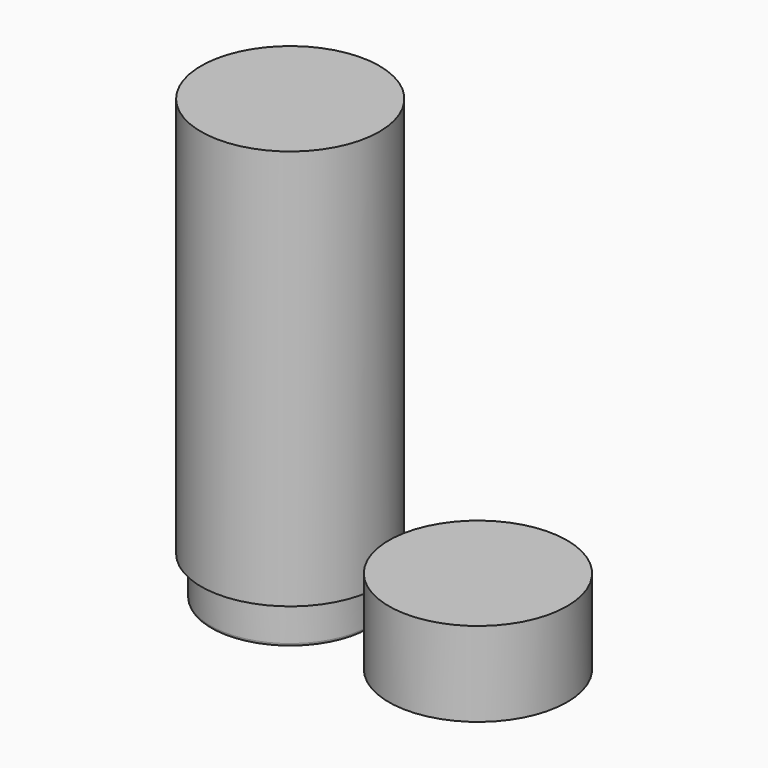
from build123d import *

# Parameters (mm, degrees)
F0_R      = 25.5
F0_R_2    = 22.5
F0_R_3    = 17.5
F1_DEPTH  = 141
F2_DEPTH  = 136
F3_DEPTH  = 66
F5_R      = 1
F6_R      = 1
F7_R      = 1
F8_R      = 28.5
F8_R_2    = 25.5
F8_R_3    = 22.5
F9_DEPTH  = 27
F10_DEPTH = 22
F11_DEPTH = 12
F12_R     = 2
F13_R     = 1
F14_R     = 28.5
F14_R_2   = 25.5
F15_DEPTH = 128


# Not quite as in the source:
# - a fillet or chamfer that OpenCascade refuses, or shapes differently, is made with other operations: its cross-section is extruded or revolved along the edge and cut away or added


with BuildPart() as f1:
    # F0 (on Top) → F1 (new body)
    with BuildSketch(Plane.XY):
        Circle(F0_R)
        Circle(F0_R_2, mode=Mode.SUBTRACT)
        Circle(F0_R_2)
        Circle(F0_R_3, mode=Mode.SUBTRACT)
        Circle(F0_R_3)
    extrude(amount=F1_DEPTH)

    # F0 (on Top) → F2 (cut)
    with BuildSketch(Plane.XY):
        Circle(F0_R_3)
    extrude(amount=F2_DEPTH, mode=Mode.SUBTRACT)

    # F0 (on Top) → F3 (cut)
    with BuildSketch(Plane.XY):
        Circle(F0_R_2)
        Circle(F0_R_3, mode=Mode.SUBTRACT)
    extrude(amount=F3_DEPTH, mode=Mode.SUBTRACT)

    # F4: fillet of radius 22.4 on 1 edges, made by hand

    # F4_s1 → F4_t2 (revolve)
    with BuildSketch(Plane.XZ):
        with BuildLine():
            ThreePointArc((22.5, 51.8932640203), (21.2130291526, 59.3765787939), (17.5, 66))
            Line((17.5, 66), (22.5, 66))
            Line((22.5, 66), (22.5, 51.8932640203))
        make_face()
    revolve(axis=Axis((0, 0, 66), (0, 0, 1)))

    # F5
    f5_edges = [f1.edges().sort_by_distance(p)[0] for p in [
        (-17.5, 0, 136),
    ]]
    fillet(f5_edges, radius=F5_R)

    # F6
    f6_edges = [f1.edges().sort_by_distance(p)[0] for p in [
        (-17.5, 0, 66),
    ]]
    fillet(f6_edges, radius=F6_R)

    # F7
    f7_edges = [f1.edges().sort_by_distance(p)[0] for p in [
        (-25.5, 0, 0),
    ]]
    fillet(f7_edges, radius=F7_R)

    # F14 (on face) → F15 (join)
    with BuildSketch(Plane.XY.offset(141)):
        Circle(F14_R)
        Circle(F14_R_2, mode=Mode.SUBTRACT)
    extrude(amount=-F15_DEPTH)


with BuildPart() as f9:
    # F8 (on Top) → F9 (new body)
    with BuildSketch(Plane.XY):
        with Locations((60, 0)):
            Circle(F8_R)
        with Locations((60, 0)):
            Circle(F8_R_2, mode=Mode.SUBTRACT)
        with Locations((60, 0)):
            Circle(F8_R_2)
        with Locations((60, 0)):
            Circle(F8_R_3, mode=Mode.SUBTRACT)
        with Locations((60, 0)):
            Circle(F8_R_3)
    extrude(amount=F9_DEPTH)

    # F8 (on Top) → F10 (cut)
    with BuildSketch(Plane.XY):
        with Locations((60, 0)):
            Circle(F8_R_3)
    extrude(amount=F10_DEPTH, mode=Mode.SUBTRACT)

    # F8 (on Top) → F11 (cut)
    with BuildSketch(Plane.XY):
        with Locations((60, 0)):
            Circle(F8_R_2)
        with Locations((60, 0)):
            Circle(F8_R_3, mode=Mode.SUBTRACT)
    extrude(amount=F11_DEPTH, mode=Mode.SUBTRACT)

    # F12
    f12_edges = [f9.edges().sort_by_distance(p)[0] for p in [
        (37.5, 0, 22),
    ]]
    fillet(f12_edges, radius=F12_R)

    # F13
    f13_edges = [f9.edges().sort_by_distance(p)[0] for p in [
        (34.5, 0, 12),
    ]]
    fillet(f13_edges, radius=F13_R)


solid = Compound([f1.part, f9.part])
